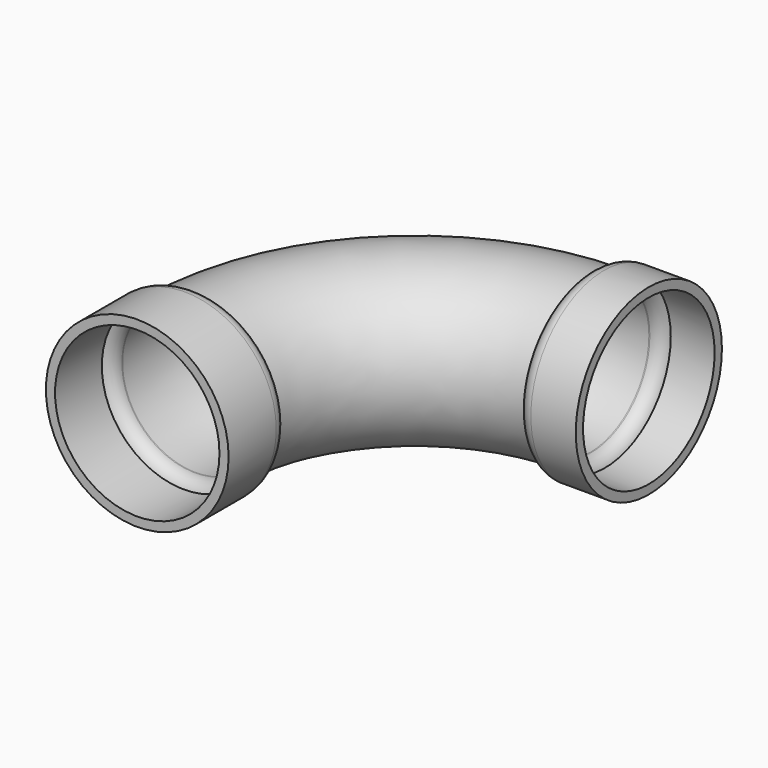
from build123d import *

# Parameters (mm, degrees)
F0_R     = 28.575
F0_R_2   = 25.4
F0_R_3   = 31.75
F3_DEPTH = 25.4
F4_DEPTH = 5.08
F5_R     = 28.575
F5_R_2   = 25.4
F6_DEPTH = 5.08
F5_R_3   = 31.75
F7_DEPTH = 20.32


# Not quite as in the source:
# - a fillet or chamfer that OpenCascade refuses, or shapes differently, is made with other operations: its cross-section is extruded or revolved along the edge and cut away or added


with BuildPart() as f2:
    # F2: sweep along a path in F1
    with BuildLine(Plane.XY) as f2_path:
        ThreePointArc((76.2, 76.2), (22.3184632736, 53.8815367264), (0, 0))
    # F0 (on Front) → F2 (sweep)
    with BuildSketch(Plane.XZ):
        Circle(F0_R)
        Circle(F0_R_2, mode=Mode.SUBTRACT)
    sweep(path=f2_path.line)

    # F0 (on Front) → F3 (join)
    with BuildSketch(Plane.XZ):
        Circle(F0_R_3)
        Circle(F0_R, mode=Mode.SUBTRACT)
    extrude(amount=F3_DEPTH)

    # F0 (on Front) → F4 (join)
    with BuildSketch(Plane.XZ):
        Circle(F0_R)
        Circle(F0_R_2, mode=Mode.SUBTRACT)
    extrude(amount=F4_DEPTH)

    # F5 (on face) → F6 (join)
    with BuildSketch(Plane.YZ.offset(76.2)):
        with Locations((76.2, 0)):
            Circle(F5_R)
        with Locations((76.2, 0)):
            Circle(F5_R_2, mode=Mode.SUBTRACT)
    extrude(amount=F6_DEPTH)

    # F5 (on face) → F7 (join)
    with BuildSketch(Plane.YZ.offset(76.2)):
        with Locations((76.2, 0)):
            Circle(F5_R_3)
        with Locations((76.2, 0)):
            Circle(F5_R, mode=Mode.SUBTRACT)
    extrude(amount=F7_DEPTH)

    # F8: fillet of radius 5.08 on 4 edges, made by hand

    # F8_s1 → F8_t2 (revolve, cut)
    with BuildSketch(Plane.XY):
        with BuildLine():
            ThreePointArc((76.5707139607, 101.6), (79.4105202921, 102.4678865162), (81.28, 104.775))
            Line((81.28, 104.775), (81.28, 101.6))
            Line((81.28, 101.6), (76.5707139607, 101.6))
        make_face()
    revolve(axis=Axis((81.28, 76.2, 0), (1, 0, 0)), mode=Mode.SUBTRACT)

    # F8_s3 → F8_t4 (revolve, cut)
    with BuildSketch(Plane.XY):
        with BuildLine():
            ThreePointArc((80.9092860393, 107.95), (78.0694797079, 107.0821134838), (76.2, 104.775))
            Line((76.2, 104.775), (76.2, 107.95))
            Line((76.2, 107.95), (80.9092860393, 107.95))
        make_face()
    revolve(axis=Axis((76.2, 76.2, 0), (1, 0, 0)), mode=Mode.SUBTRACT)

    # F8_s5 → F8_t6 (revolve, cut)
    with BuildSketch(Plane.XY):
        with BuildLine():
            ThreePointArc((28.575, -5.08), (26.2678865162, -3.2105202921), (25.4, -0.3707139607))
            Line((25.4, -0.3707139607), (25.4, -5.08))
            Line((25.4, -5.08), (28.575, -5.08))
        make_face()
    revolve(axis=Axis((0, -5.08, 0), (0, -1, 0)), mode=Mode.SUBTRACT)

    # F8_s7 → F8_t8 (revolve, cut)
    with BuildSketch(Plane.XY):
        with BuildLine():
            ThreePointArc((28.575, 0), (30.8821134838, -1.8694797079), (31.75, -4.7092860393))
            Line((31.75, -4.7092860393), (31.75, 0))
            Line((31.75, 0), (28.575, 0))
        make_face()
    revolve(axis=Axis((0, 0, 0), (0, -1, 0)), mode=Mode.SUBTRACT)


solid = f2.part
